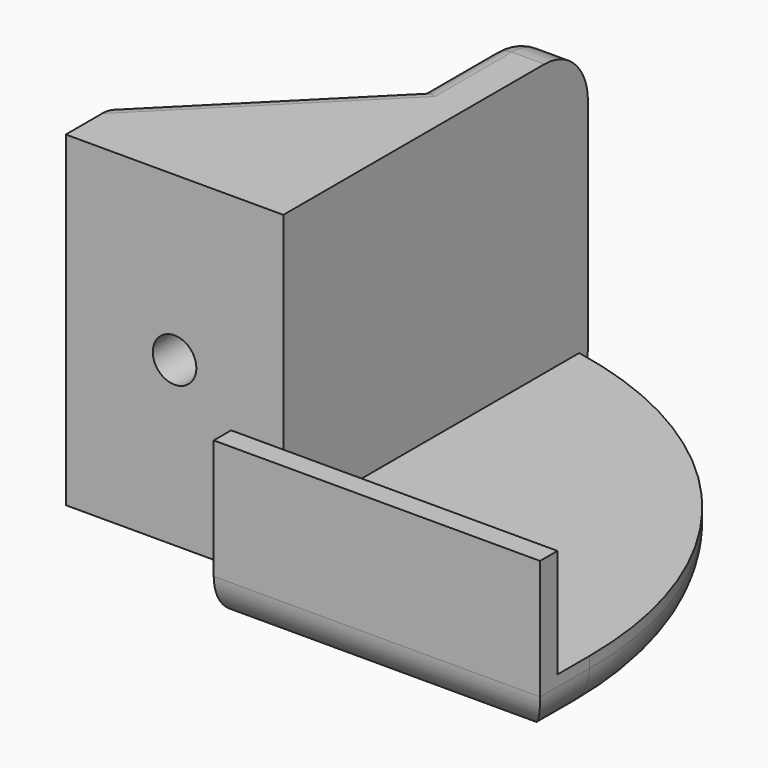
from build123d import *

# Parameters (mm, degrees)
F0_W          = 30
F0_H          = 42
F1_DEPTH      = 5
F2_T1_DEPTH   = 186.6590212458
F3_W          = 30
F3_H          = 2
F4_DEPTH      = 10
F5_W          = 35
F5_H          = 30
F6_DEPTH      = 5
F7_W          = 7
F7_H          = 30
F8_DEPTH      = 15
F9_R          = 2
F10_DEPTH     = 10
F11_R         = 4
F12_W         = 15
F12_H         = 14
F13_DEPTH     = 5
F14_W         = 15
F14_H         = 15
F15_DEPTH     = 5
F16_T4_DEPTH  = 35.8601958556
F16_T9_DEPTH  = 35.8601958556
F17_R         = 5
F18_T1_DEPTH  = 20
F18_T6_DEPTH  = 9.5699020722
F18_T11_DEPTH = 31.2132034356
F18_T16_DEPTH = 31.2132034356
F18_T21_DEPTH = 14
F18_T24_ANGLE = 90
F18_T26_ANGLE = 90
F18_T30_DEPTH = 13
F18_T36_DEPTH = 14
F18_T40_DEPTH = 31.2132034356
F18_T47_DEPTH = 13
F18_T51_DEPTH = 31.2132034356


# Not quite as in the source:
# - a fillet or chamfer that OpenCascade refuses, or shapes differently, is made with other operations: its cross-section is extruded or revolved along the edge and cut away or added


with BuildPart() as f1:
    # F0 (on Top) → F1 (new body)
    with BuildSketch(Plane.XY):
        with Locations((15, 21)):
            Rectangle(F0_W, F0_H)
    extrude(amount=F1_DEPTH)

    # F2: fillet of radius 37 on 1 edges, made by hand

    # F2_s2 → F2_t1 (cut)
    with BuildSketch(Plane.XY.offset(-90.8295106229)):
        with BuildLine():
            ThreePointArc((30, 5.6681957508), (21.5306852354, 29.2266337296), (0, 42))
            Line((0, 42), (30, 42))
            Line((30, 42), (30, 5.6681957508))
        make_face()
    extrude(amount=F2_T1_DEPTH, mode=Mode.SUBTRACT)

    # F3 (on face) → F4 (join)
    with BuildSketch(Plane.XY.offset(5)):
        with Locations((15, 1)):
            Rectangle(F3_W, F3_H)
    extrude(amount=F4_DEPTH)

    # F5 (on face) → F6 (join)
    with BuildSketch(Plane(origin=(0, 0, 0), x_dir=(0, -1, 0), z_dir=(-1, 0, 0))):
        with Locations((-25.5, 15)):
            Rectangle(F5_W, F5_H)
    extrude(amount=F6_DEPTH)

    # F7 (on face) → F8 (join)
    with BuildSketch(Plane(origin=(-5, 0, 0), x_dir=(0, -1, 0), z_dir=(-1, 0, 0))):
        with Locations((-11.5, 15)):
            Rectangle(F7_W, F7_H)
    extrude(amount=F8_DEPTH)

    # F9 (on face) → F10 (cut)
    with BuildSketch(Plane(origin=(0, 15, 0), x_dir=(-1, 0, 0), z_dir=(0, 1, 0))):
        with Locations((10, 15)):
            Circle(F9_R)
    extrude(amount=-F10_DEPTH, mode=Mode.SUBTRACT)

    # F11
    f11_edges = [f1.edges().sort_by_distance(p)[0] for p in [
        (21.530685, 29.226634, 0),
        (15, 0, 0),
    ]]
    fillet(f11_edges, radius=F11_R)

    # F12 (on face) → F13 (join)
    with BuildSketch(Plane(origin=(0, 0, 0), x_dir=(1, 0, 0), z_dir=(0, 0, -1))):
        with Locations((-12.5, -22)):
            Rectangle(F12_W, F12_H)
    extrude(amount=-F13_DEPTH)

    # F14 (on face) → F15 (join)
    with BuildSketch(Plane.XY.offset(30)):
        with Locations((-12.5, 22.5)):
            Rectangle(F14_W, F14_H)
    extrude(amount=-F15_DEPTH)

    # F16: chamfer of 15 on 2 edges, made by hand


with BuildPart() as f16_tool2:
    # F16_s3 → F16_t4 (new body)
    with BuildSketch(Plane.XY.offset(45.4300979278)):
        with BuildLine():
            Line((-20.4242640687, 14.5757359313), (-4.5757359313, 30.4242640687))
            Line((-4.5757359313, 30.4242640687), (-4.5757359313, 30.7242640687))
            ThreePointArc((-4.5757359313, 30.7242640687), (-12.2878679656, 30.3), (-20, 30.3))
            Line((-20, 30.3), (-20.3, 30))
            ThreePointArc((-20.3, 30), (-20.3, 22.2878679656), (-20.7242640687, 14.5757359313))
            Line((-20.7242640687, 14.5757359313), (-20.4242640687, 14.5757359313))
        make_face()
    extrude(amount=-F16_T4_DEPTH)

    split(bisect_by=Plane.YZ.offset(-5), keep=Keep.BOTTOM)


with BuildPart() as f1_1:
    add(f1.part)

    # F16_t1: cut F16_tool2
    add(f16_tool2.part, mode=Mode.SUBTRACT)


with BuildPart() as f16_tool7:
    # F16_s8 → F16_t9 (new body)
    with BuildSketch(Plane.XY.offset(-15.4300979278)):
        with BuildLine():
            Line((-4.5757359313, 29.4242640687), (-20.4242640687, 13.5757359313))
            Line((-20.4242640687, 13.5757359313), (-20.7242640687, 13.5757359313))
            ThreePointArc((-20.7242640687, 13.5757359313), (-20.3, 21.2878679656), (-20.3, 29))
            Line((-20.3, 29), (-20, 29.3))
            ThreePointArc((-20, 29.3), (-12.2878679656, 29.3), (-4.5757359313, 29.7242640687))
            Line((-4.5757359313, 29.7242640687), (-4.5757359313, 29.4242640687))
        make_face()
    extrude(amount=F16_T9_DEPTH)

    split(bisect_by=Plane.YZ.offset(-5), keep=Keep.BOTTOM)


with BuildPart() as f1_2:
    add(f1_1.part)

    # F16_t6: cut F16_tool7
    add(f16_tool7.part, mode=Mode.SUBTRACT)

    # F17
    f17_edges = [f1_2.edges().sort_by_distance(p)[0] for p in [
        (-2.5, 43, 0),
        (-2.5, 43, 30),
    ]]
    fillet(f17_edges, radius=F17_R)

    # F18: fillet of radius 2 on 9 edges, made by hand

    # F18_s2 → F18_t1 (cut)
    with BuildSketch(Plane.XY.offset(5)):
        with BuildLine():
            ThreePointArc((-3, 43), (-4.4142135624, 42.4142135624), (-5, 41))
            Line((-5, 41), (-5, 43))
            Line((-5, 43), (-3, 43))
        make_face()
    extrude(amount=F18_T1_DEPTH, mode=Mode.SUBTRACT)


with BuildPart() as f18_tool4:
    # F18_s5 → F18_t6 (new body)
    with BuildSketch(Plane.XY.offset(25)):
        with BuildLine():
            ThreePointArc((-20, 13), (-19.4142135624, 14.4142135624), (-18, 15))
            Line((-18, 15), (-20, 15))
            Line((-20, 15), (-20, 13))
        make_face()
    extrude(amount=-F18_T6_DEPTH)

    split(bisect_by=Plane(origin=(-17, 17, 0), x_dir=(0, 0, 1), z_dir=(-0.7071067812, 0.7071067812, 0)), keep=Keep.TOP)


with BuildPart() as f1_3:
    add(f1_2.part)

    # F18_t3: cut F18_tool4
    add(f18_tool4.part, mode=Mode.SUBTRACT)


with BuildPart() as f18_tool9:
    # F18_s10 → F18_t11 (new body)
    with BuildSketch(Plane(origin=(-6.5355339059, -6.5355339059, 0), x_dir=(0, 0, 1), z_dir=(0.7071067812, 0.7071067812, 0))):
        with BuildLine():
            ThreePointArc((0, -22.0416305603), (0.5857864376, -23.4558441227), (2, -24.0416305603))
            Line((2, -24.0416305603), (0, -24.0416305603))
            Line((0, -24.0416305603), (0, -22.0416305603))
        make_face()
    extrude(amount=F18_T11_DEPTH)

    split(bisect_by=Plane.YZ.offset(-5), keep=Keep.BOTTOM)


with BuildPart() as f1_4:
    add(f1_3.part)

    # F18_t8: cut F18_tool9
    add(f18_tool9.part, mode=Mode.SUBTRACT)


with BuildPart() as f18_tool14:
    # F18_s15 → F18_t16 (new body)
    with BuildSketch(Plane(origin=(16.0355339059, 16.0355339059, 0), x_dir=(0, 0, 1), z_dir=(-0.7071067812, -0.7071067812, 0))):
        with BuildLine():
            ThreePointArc((30, 22.7487373415), (29.4142135624, 24.1629509039), (28, 24.7487373415))
            Line((28, 24.7487373415), (30, 24.7487373415))
            Line((30, 24.7487373415), (30, 22.7487373415))
        make_face()
    extrude(amount=F18_T16_DEPTH)

    split(bisect_by=Plane.YZ.offset(-5), keep=Keep.BOTTOM)


with BuildPart() as f1_5:
    add(f1_4.part)

    # F18_t13: cut F18_tool14
    add(f18_tool14.part, mode=Mode.SUBTRACT)


with BuildPart() as f18_tool19:
    # F18_s20 → F18_t21 (new body)
    with BuildSketch(Plane.XZ.offset(-24)):
        with BuildLine():
            ThreePointArc((-3, 0), (-4.4142135624, 0.5857864376), (-5, 2))
            Line((-5, 2), (-5, 0))
            Line((-5, 0), (-3, 0))
        make_face()
    extrude(amount=-F18_T21_DEPTH)

    split(bisect_by=Plane(origin=(-17, 17, 0), x_dir=(0, 0, 1), z_dir=(-0.7071067812, 0.7071067812, 0)), keep=Keep.TOP)


with BuildPart() as f1_6:
    add(f1_5.part)

    # F18_t18: cut F18_tool19
    add(f18_tool19.part, mode=Mode.SUBTRACT)

    # F18_s23 → F18_t24 (revolve, cut)
    with BuildSketch(Plane.XY.offset(5)):
        with BuildLine():
            ThreePointArc((-3, 43), (-4.4142135624, 42.4142135624), (-5, 41))
            Line((-5, 41), (-5, 43))
            Line((-5, 43), (-3, 43))
        make_face()
    revolve(axis=Axis((-5, 38, 5), (-1, 0, 0)), revolution_arc=F18_T24_ANGLE, mode=Mode.SUBTRACT)

    # F18_s25 → F18_t26 (revolve, cut)
    with BuildSketch(Plane.XY.offset(25)):
        with BuildLine():
            ThreePointArc((-3, 43), (-4.4142135624, 42.4142135624), (-5, 41))
            Line((-5, 41), (-5, 43))
            Line((-5, 43), (-3, 43))
        make_face()
    revolve(axis=Axis((-5, 38, 25), (1, 0, 0)), revolution_arc=F18_T26_ANGLE, mode=Mode.SUBTRACT)


with BuildPart() as f18_tool28:
    # F18_s29 → F18_t30 (new body)
    with BuildSketch(Plane.XZ.offset(-25)):
        with BuildLine():
            ThreePointArc((-3, 30), (-4.4142135624, 29.4142135624), (-5, 28))
            Line((-5, 28), (-5, 30))
            Line((-5, 30), (-3, 30))
        make_face()
    extrude(amount=-F18_T30_DEPTH)

    split(bisect_by=Plane(origin=(-17.5, 17.5, 0), x_dir=(0, 0, 1), z_dir=(-0.7071067812, 0.7071067812, 0)), keep=Keep.TOP)


with BuildPart() as f1_7:
    add(f1_6.part)

    # F18_t27: cut F18_tool28
    add(f18_tool28.part, mode=Mode.SUBTRACT)


with BuildPart() as f18_tool34:
    # F18_s35 → F18_t36 (new body)
    with BuildSketch(Plane.XZ.offset(-24)):
        with BuildLine():
            ThreePointArc((-3, 0), (-4.4142135624, 0.5857864376), (-5, 2))
            Line((-5, 2), (-5, 0))
            Line((-5, 0), (-3, 0))
        make_face()
    extrude(amount=-F18_T36_DEPTH)

    split(bisect_by=Plane(origin=(-17, 17, 0), x_dir=(0, 0, 1), z_dir=(0.7071067812, -0.7071067812, 0)), keep=Keep.TOP)


with BuildPart() as f18_tool38:
    # F18_s39 → F18_t40 (new body)
    with BuildSketch(Plane(origin=(-6.5355339059, -6.5355339059, 0), x_dir=(0, 0, 1), z_dir=(0.7071067812, 0.7071067812, 0))):
        with BuildLine():
            ThreePointArc((0, -22.0416305603), (0.5857864376, -23.4558441227), (2, -24.0416305603))
            Line((2, -24.0416305603), (0, -24.0416305603))
            Line((0, -24.0416305603), (0, -22.0416305603))
        make_face()
    extrude(amount=F18_T40_DEPTH)

    split(bisect_by=Plane.YZ.offset(-5), keep=Keep.TOP)


with BuildPart() as f18_tool34_1:
    add(f18_tool34.part)

    # F18_t42: intersect F18_tool38
    add(f18_tool38.part, mode=Mode.INTERSECT)


with BuildPart() as f1_8:
    add(f1_7.part)

    # F18_t32: cut F18_tool34
    add(f18_tool34_1.part, mode=Mode.SUBTRACT)


with BuildPart() as f18_tool45:
    # F18_s46 → F18_t47 (new body)
    with BuildSketch(Plane.XZ.offset(-25)):
        with BuildLine():
            ThreePointArc((-3, 30), (-4.4142135624, 29.4142135624), (-5, 28))
            Line((-5, 28), (-5, 30))
            Line((-5, 30), (-3, 30))
        make_face()
    extrude(amount=-F18_T47_DEPTH)

    split(bisect_by=Plane(origin=(-17.5, 17.5, 0), x_dir=(0, 0, 1), z_dir=(0.7071067812, -0.7071067812, 0)), keep=Keep.TOP)


with BuildPart() as f18_tool49:
    # F18_s50 → F18_t51 (new body)
    with BuildSketch(Plane(origin=(16.0355339059, 16.0355339059, 0), x_dir=(0, 0, 1), z_dir=(-0.7071067812, -0.7071067812, 0))):
        with BuildLine():
            ThreePointArc((30, 22.7487373415), (29.4142135624, 24.1629509039), (28, 24.7487373415))
            Line((28, 24.7487373415), (30, 24.7487373415))
            Line((30, 24.7487373415), (30, 22.7487373415))
        make_face()
    extrude(amount=F18_T51_DEPTH)

    split(bisect_by=Plane.YZ.offset(-5), keep=Keep.TOP)


with BuildPart() as f18_tool45_1:
    add(f18_tool45.part)

    # F18_t53: intersect F18_tool49
    add(f18_tool49.part, mode=Mode.INTERSECT)


with BuildPart() as f1_9:
    add(f1_8.part)

    # F18_t43: cut F18_tool45
    add(f18_tool45_1.part, mode=Mode.SUBTRACT)


solid = f1_9.part
